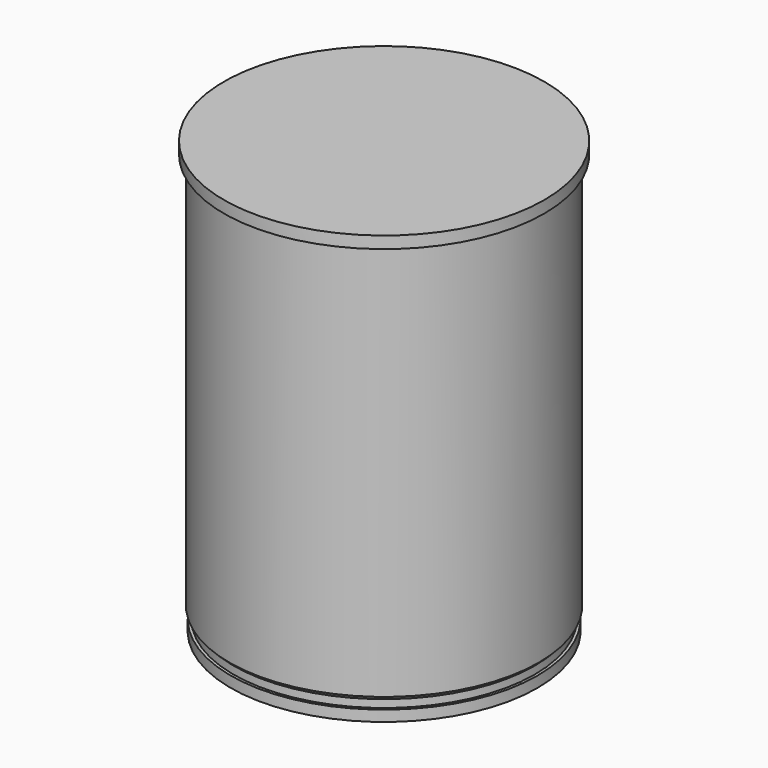
from build123d import *

# Parameters (mm, degrees)
F0_R        = 35.8775
F1_DEPTH    = 2.54
F2_R        = 35.21075
F3_DEPTH    = 1.778
F4_R        = 36.195
F5_DEPTH    = 93.853
F6_R        = 37.465
F7_DEPTH    = 2.794
F8_S5_R     = 35.21075
F8_T6_DEPTH = 53


# Not quite as in the source:
# - a fillet or chamfer that OpenCascade refuses, or shapes differently, is made with other operations: its cross-section is extruded or revolved along the edge and cut away or added


with BuildPart() as f1:
    # F0 (on Top) → F1 (new body)
    with BuildSketch(Plane.XY):
        Circle(F0_R)
    extrude(amount=F1_DEPTH)

    # F2 (on face) → F3 (join)
    with BuildSketch(Plane.XY.offset(2.54)):
        Circle(F2_R)
    extrude(amount=F3_DEPTH)

    # F4 (on face) → F5 (join)
    with BuildSketch(Plane.XY.offset(4.318)):
        Circle(F4_R)
    extrude(amount=F5_DEPTH)

    # F6 (on face) → F7 (join)
    with BuildSketch(Plane.XY.offset(98.171)):
        Circle(F6_R)
    extrude(amount=F7_DEPTH)

    # F8: chamfer of 1.016 on 1 edges, made by hand


with BuildPart() as f8_tool2:
    # F8_s3 → F8_t4 (revolve)
    with BuildSketch(Plane.XZ):
        Polygon((36.195, 5.334), (35.179, 4.318), (36.195, 4.318), align=None)
    revolve(axis=Axis((0, 0, 4.318), (0, 0, 1)))

    # F8_s5 → F8_t6 (cut, symmetric)
    with BuildSketch(Plane.XY.offset(4.8)):
        Circle(F8_S5_R)
    extrude(amount=F8_T6_DEPTH, both=True, mode=Mode.SUBTRACT)


with BuildPart() as f1_1:
    add(f1.part)

    # F8_t1: cut F8_tool2
    add(f8_tool2.part, mode=Mode.SUBTRACT)


solid = f1_1.part
